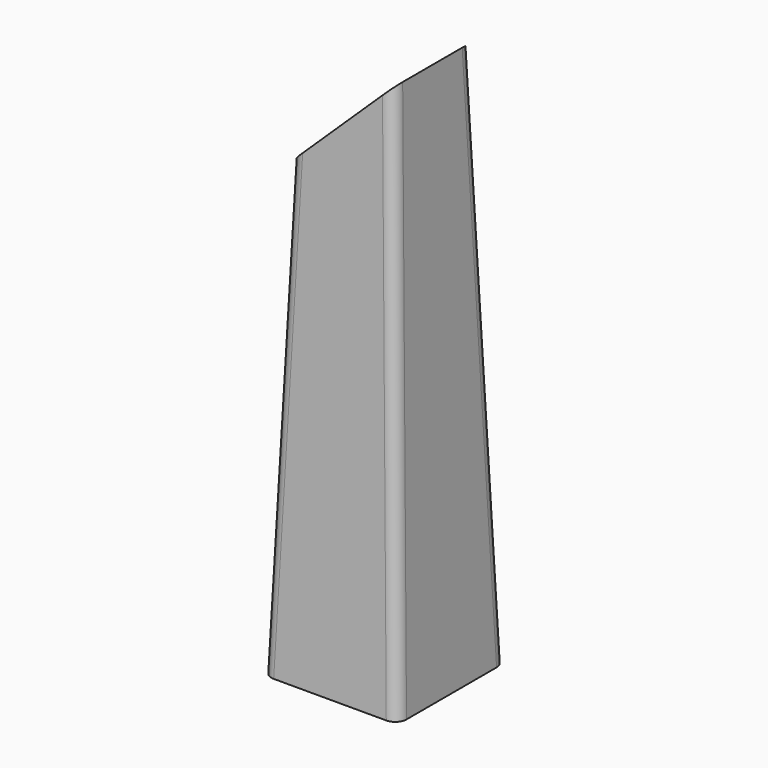
from build123d import *

# Parameters (mm, degrees)
F2_DEPTH    = 520
F2_TAPER    = 2
F3_T1_DEPTH = 701.1716597564
F4_R        = 10
F5_T        = -2.5


# Not quite as in the source:
# - a fillet or chamfer that OpenCascade refuses, or shapes differently, is made with other operations: its cross-section is extruded or revolved along the edge and cut away or added


with BuildPart() as f2:
    # F0 (on Top) → F2 (new body)
    with BuildSketch(Plane.XY):
        Polygon((120, 120), (0, 120), (60, 60), align=None)
        Polygon((60, 60), (120, 0), (120, 120), align=None)
        Polygon((60, 60), (0, 0), (120, 0), align=None)
        Polygon((0, 120), (0, 0), (60, 60), align=None)
    extrude(amount=F2_DEPTH, taper=F2_TAPER)

    # F3: chamfer of 120 on 1 edges, made by hand

    # F3_s2 → F3_t1 (cut)
    with BuildSketch(Plane.XZ.offset(-410.5858298782)):
        Polygon((13.9708605314, 400.0731007577), (138.1588001357, 520), (18.1588001357, 520), align=None)
    extrude(amount=F3_T1_DEPTH, mode=Mode.SUBTRACT)

    # F4
    f4_edges = [f2.edges().sort_by_distance(p)[0] for p in [
        (6.98543, 6.98543, 200.03655),
        (6.98543, 113.01457, 200.03655),
        (111.512985, 8.487015, 243.03631),
        (111.512985, 111.512985, 243.03631),
    ]]
    fillet(f4_edges, radius=F4_R)

    # F5
    f5_openings = [f2.faces().sort_by_distance(p)[0] for p in [
        (60, 60, 0),
    ]]
    offset(amount=F5_T, openings=f5_openings)


solid = f2.part
